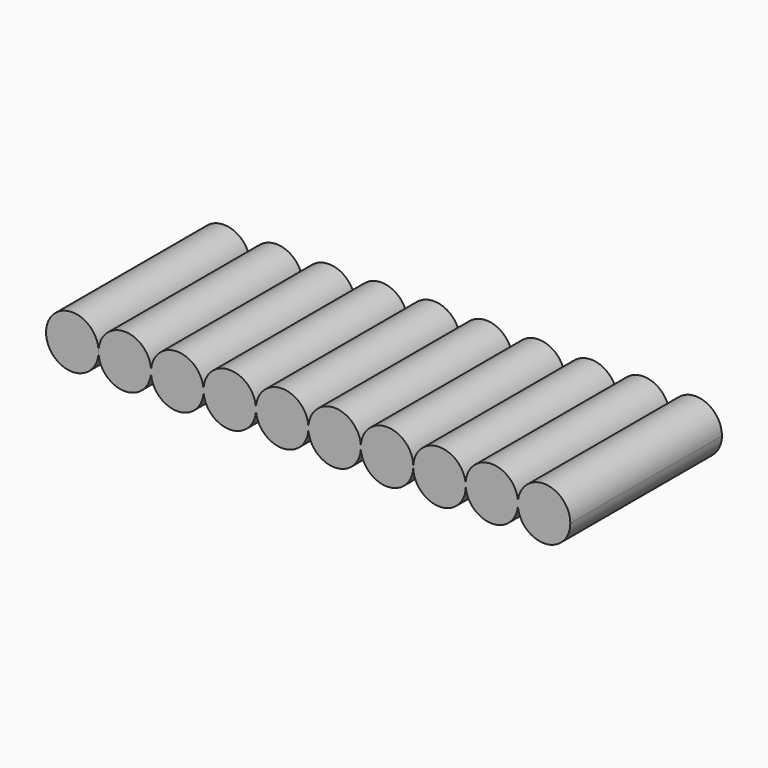
from build123d import *

# Parameters (mm, degrees)
F0_R     = 9.0043
F1_DEPTH = 65
F2_DEPTH = 65


with BuildPart() as f1:
    # F0 (on Front) → F1 (new body)
    with BuildSketch(Plane.XZ):
        Circle(F0_R)
    extrude(amount=F1_DEPTH)


with BuildPart() as f1b:
    # F0 (on Front) → F1, piece 2 (new body)
    with BuildSketch(Plane.XZ):
        with BuildLine():
            ThreePointArc((27.0043, 0), (18.0043, 9), (9.0043, 0))
            ThreePointArc((9.0043, 0), (17.9190098256, -8.9995958568), (27.0026834636, -0.1705726889))
            ThreePointArc((27.0026834636, -0.1705726889), (27.0030876068, -0.0852825145), (27.0043, 0))
        make_face()
    extrude(amount=F1_DEPTH)


with BuildPart() as f1c:
    # F0 (on Front) → F1, piece 3 (new body)
    with BuildSketch(Plane.XZ):
        with BuildLine():
            ThreePointArc((45.0013565478, -0.0160323255), (36.0107009342, 8.82942374), (27.0043, 0))
            ThreePointArc((27.0043, 0), (27.0038958568, -0.0852901744), (27.0026834636, -0.1705726889))
            ThreePointArc((27.0026834636, -0.1705726889), (36.0026834636, -9.1705726889), (45.0026834636, -0.1705726889))
            ThreePointArc((45.0026834636, -0.1705726889), (45.0023517285, -0.0932996589), (45.0013565478, -0.0160323255))
        make_face()
        with BuildLine():
            ThreePointArc((62.9929668109, 0.4942702989), (53.7448335524, 9.1348895724), (45.0013279832, -0.016032816))
            ThreePointArc((45.0013279832, -0.016032816), (54.008018538, -8.8614888815), (62.9989352075, 0))
            ThreePointArc((62.9989352075, 0), (62.9925570229, 0.2470941665), (62.9929668109, 0.4942702989))
        make_face()
    extrude(amount=F1_DEPTH)


with BuildPart() as f1d:
    # F0 (on Front) → F1, piece 4 (new body)
    with BuildSketch(Plane.XZ):
        with BuildLine():
            ThreePointArc((80.9834577198, 0.745515077), (71.8662244177, 9.3548852314), (62.9929668109, 0.4942702989))
            ThreePointArc((62.9929668109, 0.4942702989), (62.9982423314, 0.3164236907), (63.0000010674, 0.1385075474))
            ThreePointArc((63.0000010674, 0.1385075474), (62.9997345985, 0.0692517232), (62.9989352075, 0))
            ThreePointArc((62.9989352075, 0), (71.9919009511, -8.6442372485), (80.9848666946, 0))
            ThreePointArc((80.9848666946, 0), (80.9764395366, 0.3727429432), (80.9834577198, 0.745515077))
        make_face()
    extrude(amount=F1_DEPTH)


with BuildPart() as f1e:
    # F0 (on Front) → F1, piece 5 (new body)
    with BuildSketch(Plane.XZ):
        with BuildLine():
            ThreePointArc((98.9644590085, 0.8536672309), (89.9222912288, 9.3895895297), (80.9834577198, 0.745515077))
            ThreePointArc((80.9834577198, 0.745515077), (80.9897898957, 0.5506846354), (80.9919009511, 0.3557627515))
            ThreePointArc((80.9919009511, 0.3557627515), (80.9901422151, 0.1778466082), (80.9848666946, 0))
            ThreePointArc((80.9848666946, 0), (89.9764234633, -8.6102476745), (98.967980232, 0))
            ThreePointArc((98.967980232, 0), (98.9560923398, 0.4267918422), (98.9644590085, 0.8536672309))
        make_face()
    extrude(amount=F1_DEPTH)


with BuildPart() as f2:
    # F0 (on Front) → F2 (new body)
    with BuildSketch(Plane.XZ):
        Circle(F0_R)
    extrude(amount=F2_DEPTH)


with BuildPart() as f2b:
    # F0 (on Front) → F2, piece 2 (new body)
    with BuildSketch(Plane.XZ):
        with BuildLine():
            ThreePointArc((62.9929668109, 0.4942702989), (53.7448335524, 9.1348895724), (45.0013279832, -0.016032816))
            ThreePointArc((45.0013279832, -0.016032816), (54.008018538, -8.8614888815), (62.9989352075, 0))
            ThreePointArc((62.9989352075, 0), (62.9925570229, 0.2470941665), (62.9929668109, 0.4942702989))
        make_face()
        with BuildLine():
            ThreePointArc((27.0043, 0), (18.0043, 9), (9.0043, 0))
            ThreePointArc((9.0043, 0), (17.9190098256, -8.9995958568), (27.0026834636, -0.1705726889))
            ThreePointArc((27.0026834636, -0.1705726889), (27.0030876068, -0.0852825145), (27.0043, 0))
        make_face()
        with BuildLine():
            ThreePointArc((45.0013565478, -0.0160323255), (36.0107009342, 8.82942374), (27.0043, 0))
            ThreePointArc((27.0043, 0), (27.0038958568, -0.0852901744), (27.0026834636, -0.1705726889))
            ThreePointArc((27.0026834636, -0.1705726889), (36.0026834636, -9.1705726889), (45.0026834636, -0.1705726889))
            ThreePointArc((45.0026834636, -0.1705726889), (45.0023517285, -0.0932996589), (45.0013565478, -0.0160323255))
        make_face()
        with BuildLine():
            ThreePointArc((27.0026834636, -0.1705726889), (27.0038958568, -0.0852901744), (27.0043, 0))
            ThreePointArc((27.0043, 0), (27.0030876068, -0.0852825145), (27.0026834636, -0.1705726889))
        make_face()
        with BuildLine():
            ThreePointArc((80.9834577198, 0.745515077), (71.8662244177, 9.3548852314), (62.9929668109, 0.4942702989))
            ThreePointArc((62.9929668109, 0.4942702989), (62.9982423314, 0.3164236907), (63.0000010674, 0.1385075474))
            ThreePointArc((63.0000010674, 0.1385075474), (62.9997345985, 0.0692517232), (62.9989352075, 0))
            ThreePointArc((62.9989352075, 0), (71.9919009511, -8.6442372485), (80.9848666946, 0))
            ThreePointArc((80.9848666946, 0), (80.9764395366, 0.3727429432), (80.9834577198, 0.745515077))
        make_face()
        with BuildLine():
            ThreePointArc((63.0000010674, 0.1385075474), (62.9982423314, 0.3164236907), (62.9929668109, 0.4942702989))
            ThreePointArc((62.9929668109, 0.4942702989), (62.9925570229, 0.2470941665), (62.9989352075, 0))
            ThreePointArc((62.9989352075, 0), (62.9997345985, 0.0692517232), (63.0000010674, 0.1385075474))
        make_face()
        with BuildLine():
            ThreePointArc((98.9644590085, 0.8536672309), (89.9222912288, 9.3895895297), (80.9834577198, 0.745515077))
            ThreePointArc((80.9834577198, 0.745515077), (80.9897898957, 0.5506846354), (80.9919009511, 0.3557627515))
            ThreePointArc((80.9919009511, 0.3557627515), (80.9901422151, 0.1778466082), (80.9848666946, 0))
            ThreePointArc((80.9848666946, 0), (89.9764234633, -8.6102476745), (98.967980232, 0))
            ThreePointArc((98.967980232, 0), (98.9560923398, 0.4267918422), (98.9644590085, 0.8536672309))
        make_face()
        with BuildLine():
            ThreePointArc((80.9919009511, 0.3557627515), (80.9897898957, 0.5506846354), (80.9834577198, 0.745515077))
            ThreePointArc((80.9834577198, 0.745515077), (80.9764395366, 0.3727429432), (80.9848666946, 0))
            ThreePointArc((80.9848666946, 0), (80.9901422151, 0.1778466082), (80.9919009511, 0.3557627515))
        make_face()
        with BuildLine():
            ThreePointArc((116.9524651409, 0.716697116), (108.0245445118, 9.4636540023), (98.9644590085, 0.8536672309))
            ThreePointArc((98.9644590085, 0.8536672309), (98.9734318524, 0.6217869068), (98.9764234633, 0.3897523255))
            ThreePointArc((98.9764234633, 0.3897523255), (98.9743124079, 0.1948304416), (98.967980232, 0))
            ThreePointArc((98.967980232, 0), (107.9560157772, -8.5360850946), (116.9440513223, 0))
            ThreePointArc((116.9440513223, 0), (116.9411208158, 0.3584323492), (116.9524651409, 0.716697116))
        make_face()
        with BuildLine():
            ThreePointArc((98.9764234633, 0.3897523255), (98.9734318524, 0.6217869068), (98.9644590085, 0.8536672309))
            ThreePointArc((98.9644590085, 0.8536672309), (98.9560923398, 0.4267918422), (98.967980232, 0))
            ThreePointArc((98.967980232, 0), (98.9743124079, 0.1948304416), (98.9764234633, 0.3897523255))
        make_face()
        with BuildLine():
            ThreePointArc((134.8870833011, 1.2318938033), (125.6820698577, 9.2490710848), (116.9524651409, 0.716697116))
            ThreePointArc((116.9524651409, 0.716697116), (116.9551280743, 0.5903184783), (116.9560157772, 0.4639149054))
            ThreePointArc((116.9560157772, 0.4639149054), (116.9530241662, 0.2318803241), (116.9440513223, 0))
            ThreePointArc((116.9440513223, 0), (125.940500686, -8.7472177894), (134.9369500497, 0))
            ThreePointArc((134.9369500497, 0), (134.8908973596, 0.6150919971), (134.8870833011, 1.2318938033))
        make_face()
        with BuildLine():
            ThreePointArc((116.9560157772, 0.4639149054), (116.9551280743, 0.5903184783), (116.9524651409, 0.716697116))
            ThreePointArc((116.9524651409, 0.716697116), (116.9411208158, 0.3584323492), (116.9440513223, 0))
            ThreePointArc((116.9440513223, 0), (116.9530241662, 0.2318803241), (116.9560157772, 0.4639149054))
        make_face()
        with BuildLine():
            ThreePointArc((152.8445059025, 1.8163443168), (143.5907695532, 9.9743486524), (134.8870833011, 1.2318938033))
            ThreePointArc((134.8870833011, 1.2318938033), (134.9271364174, 0.7430660386), (134.940500686, 0.2527822106))
            ThreePointArc((134.940500686, 0.2527822106), (134.9396129832, 0.1263786377), (134.9369500497, 0))
            ThreePointArc((134.9369500497, 0), (143.8835326649, -8.0208884073), (152.83011528, 0))
            ThreePointArc((152.83011528, 0), (152.7913709763, 0.908536131), (152.8445059025, 1.8163443168))
        make_face()
        with BuildLine():
            ThreePointArc((134.940500686, 0.2527822106), (134.9271364174, 0.7430660386), (134.8870833011, 1.2318938033))
            ThreePointArc((134.8870833011, 1.2318938033), (134.8908973596, 0.6150919971), (134.9369500497, 0))
            ThreePointArc((134.9369500497, 0), (134.9396129832, 0.1263786377), (134.940500686, 0.2527822106))
        make_face()
        with BuildLine():
            ThreePointArc((170.7910885176, 0.8372327241), (162.2813723456, 9.8238684555), (152.8445059025, 1.8163443168))
            ThreePointArc((152.8445059025, 1.8163443168), (152.87377068, 1.3981825063), (152.8835326649, 0.9791115927))
            ThreePointArc((152.8835326649, 0.9791115927), (152.8701683962, 0.4888277647), (152.83011528, 0))
            ThreePointArc((152.83011528, 0), (162.2101594312, -8.1530052911), (170.7910885176, 0.8372327241))
        make_face()
        with BuildLine():
            ThreePointArc((152.8835326649, 0.9791115927), (152.87377068, 1.3981825063), (152.8445059025, 1.8163443168))
            ThreePointArc((152.8445059025, 1.8163443168), (152.7913709763, 0.908536131), (152.83011528, 0))
            ThreePointArc((152.83011528, 0), (152.8701683962, 0.4888277647), (152.8835326649, 0.9791115927))
        make_face()
    extrude(amount=F2_DEPTH)


solid = Compound([f1.part, f1b.part, f1c.part, f1d.part, f1e.part, f2.part, f2b.part])
